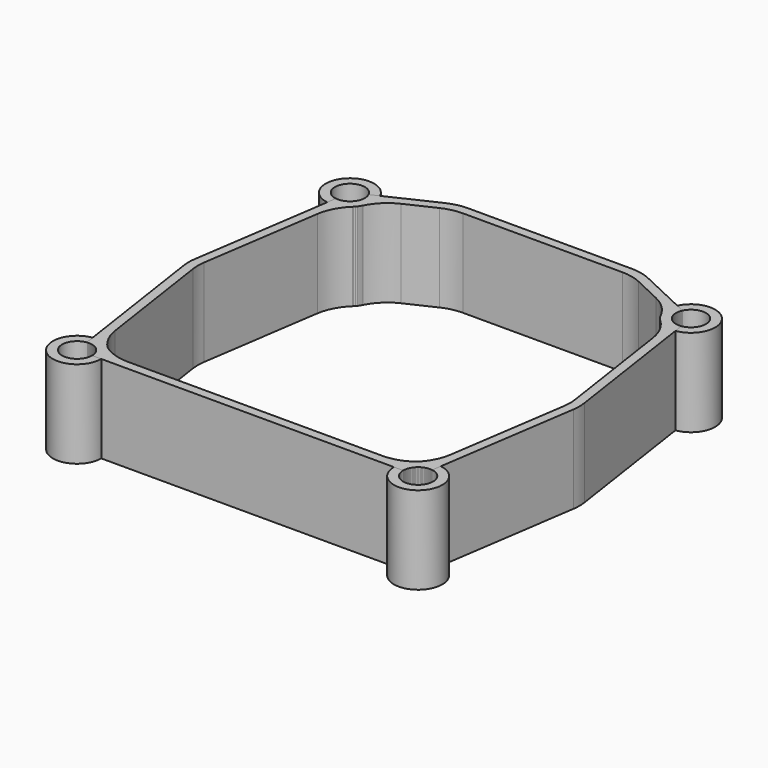
from build123d import *

# Parameters (mm, degrees)
F0_R        = 5.25
F1_DEPTH    = 19
F3_DEPTH    = 19
F4_R        = 3.25
F5_DEPTH    = 25
F7_DEPTH    = 25
F8_T1_DEPTH = 19
F8_T3_DEPTH = 26.4324324324
F8_T5_DEPTH = 30.1768389253


# Not quite as in the source:
# - a fillet or chamfer that OpenCascade refuses, or shapes differently, is made with other operations: its cross-section is extruded or revolved along the edge and cut away or added


with BuildPart() as f1:
    # F0 (on Top) → F1 (new body)
    with BuildSketch(Plane.XY):
        with Locations((-37, 37)):
            Circle(F0_R)
    extrude(amount=F1_DEPTH)


with BuildPart() as f1b:
    # F0 (on Top) → F1, piece 2 (new body)
    with BuildSketch(Plane.XY):
        with Locations((37, 37)):
            Circle(F0_R)
    extrude(amount=F1_DEPTH)


with BuildPart() as f1c:
    # F0 (on Top) → F1, piece 3 (new body)
    with BuildSketch(Plane.XY):
        with Locations((37, -37)):
            Circle(F0_R)
    extrude(amount=F1_DEPTH)


with BuildPart() as f1d:
    # F0 (on Top) → F1, piece 4 (new body)
    with BuildSketch(Plane.XY):
        with Locations((-37, -37)):
            Circle(F0_R)
    extrude(amount=F1_DEPTH)


with BuildPart() as f3:
    # F2 (on Top) → F3 (new body)
    with BuildSketch(Plane.XY):
        Polygon((20, 45), (-20, 45), (-37, 37), (-42.5, 0), (-37, -37), (37, -37), (42.5, 0), (37, 37), align=None)
    extrude(amount=F3_DEPTH)


with BuildPart() as f5_tool:
    # F4 (on Top) → F5 (new body)
    with BuildSketch(Plane.XY):
        with Locations((-37, 37)):
            Circle(F4_R)
        with Locations((37, 37)):
            Circle(F4_R)
        with Locations((37, -37)):
            Circle(F4_R)
        with Locations((-37, -37)):
            Circle(F4_R)
    extrude(amount=F5_DEPTH)


with BuildPart() as f1_1:
    add(f1.part)

    # F5: cut by f5_tool
    add(f5_tool.part, mode=Mode.SUBTRACT)


with BuildPart() as f1b_1:
    add(f1b.part)

    # F5: cut by f5_tool
    add(f5_tool.part, mode=Mode.SUBTRACT)


with BuildPart() as f1c_1:
    add(f1c.part)

    # F5: cut by f5_tool
    add(f5_tool.part, mode=Mode.SUBTRACT)


with BuildPart() as f1d_1:
    add(f1d.part)

    # F5: cut by f5_tool
    add(f5_tool.part, mode=Mode.SUBTRACT)


with BuildPart() as f3_1:
    add(f3.part)

    # F5: cut by f5_tool
    add(f5_tool.part, mode=Mode.SUBTRACT)

    # F6 (on Top) → F7 (cut)
    with BuildSketch(Plane.XY):
        with BuildLine():
            Line((19.552926443, 43), (-19.552926443, 43))
            Line((-19.552926443, 43), (-31.7563055954, 37.25723334))
            ThreePointArc((-31.7563055954, 37.25723334), (-32.7866811629, 33.8678371088), (-35.7354533115, 31.9045685489))
            Line((-35.7354533115, 31.9045685489), (-40.478024312, 0))
            Line((-40.478024312, 0), (-35.7354533115, -31.9045685489))
            ThreePointArc((-35.7354533115, -31.9045685489), (-33.571450675, -33.0241290858), (-32.1458780403, -35))
            Line((-32.1458780403, -35), (32.1458780403, -35))
            ThreePointArc((32.1458780403, -35), (33.571450675, -33.0241290858), (35.7354533115, -31.9045685489))
            Line((35.7354533115, -31.9045685489), (40.478024312, 0))
            Line((40.478024312, 0), (35.7354533115, 31.9045685489))
            ThreePointArc((35.7354533115, 31.9045685489), (32.7866811629, 33.8678371088), (31.7563055954, 37.25723334))
            Line((31.7563055954, 37.25723334), (19.552926443, 43))
        make_face()
    extrude(amount=F7_DEPTH, mode=Mode.SUBTRACT)

    # F8: fillet of radius 10 on 16 edges, made by hand

    # F8_s2 → F8_t1 (join)
    with BuildSketch(Plane.XY):
        with BuildLine():
            ThreePointArc((21.5755290212, 42.048187022), (19.4990867668, 42.7591462285), (17.3175586579, 43))
            Line((17.3175586579, 43), (19.552926443, 43))
            Line((19.552926443, 43), (21.5755290212, 42.048187022))
        make_face()
        with BuildLine():
            ThreePointArc((-17.3175586579, 43), (-19.4990867668, 42.7591462285), (-21.5755290212, 42.048187022))
            Line((-21.5755290212, 42.048187022), (-19.552926443, 43))
            Line((-19.552926443, 43), (-17.3175586579, 43))
        make_face()
        with BuildLine():
            ThreePointArc((-40.2594616371, 1.4703307219), (-40.3681458718, 0), (-40.2594616371, -1.4703307219))
            Line((-40.2594616371, -1.4703307219), (-40.478024312, 0))
            Line((-40.478024312, 0), (-40.2594616371, 1.4703307219))
        make_face()
        with BuildLine():
            ThreePointArc((40.2594616371, -1.4703307219), (40.3681458718, 0), (40.2594616371, 1.4703307219))
            Line((40.2594616371, 1.4703307219), (40.478024312, 0))
            Line((40.478024312, 0), (40.2594616371, -1.4703307219))
        make_face()
        with BuildLine():
            ThreePointArc((-33.3901050909, 33.188024299), (-35.3836316287, 30.5457403999), (-36.405430553, 27.3974489237))
            Line((-36.405430553, 27.3974489237), (-35.7354533115, 31.9045685489))
            ThreePointArc((-35.7354533115, 31.9045685489), (-34.4797103564, 32.3944989293), (-33.3901050909, 33.188024299))
        make_face()
        with BuildLine():
            ThreePointArc((-27.6333696517, 39.19743849), (-30.3537332547, 37.3118526055), (-32.3095636894, 34.6415455874))
            ThreePointArc((-32.3095636894, 34.6415455874), (-31.8636400174, 35.9135810529), (-31.7563055954, 37.25723334))
            Line((-31.7563055954, 37.25723334), (-27.6333696517, 39.19743849))
        make_face()
        with BuildLine():
            ThreePointArc((-33.3901050909, -33.188024299), (-35.3836316287, -30.5457403999), (-36.405430553, -27.3974489237))
            Line((-36.405430553, -27.3974489237), (-35.7354533115, -31.9045685489))
            ThreePointArc((-35.7354533115, -31.9045685489), (-34.4797103564, -32.3944989293), (-33.3901050909, -33.188024299))
        make_face()
        with BuildLine():
            ThreePointArc((-33.7602284039, -32.868852459), (-30.8535476338, -34.452209387), (-27.5892348876, -35))
            Line((-27.5892348876, -35), (-32.1458780403, -35))
            ThreePointArc((-32.1458780403, -35), (-32.8151193944, -33.8299409601), (-33.7602284039, -32.868852459))
        make_face()
        with BuildLine():
            ThreePointArc((36.405430553, 27.3974489237), (35.3836316287, 30.5457403999), (33.3901050909, 33.188024299))
            ThreePointArc((33.3901050909, 33.188024299), (34.4797103564, 32.3944989293), (35.7354533115, 31.9045685489))
            Line((35.7354533115, 31.9045685489), (36.405430553, 27.3974489237))
        make_face()
        with BuildLine():
            ThreePointArc((32.3095636894, 34.6415455874), (30.3537332547, 37.3118526055), (27.6333696517, 39.19743849))
            Line((27.6333696517, 39.19743849), (31.7563055954, 37.25723334))
            ThreePointArc((31.7563055954, 37.25723334), (31.8636400174, 35.9135810529), (32.3095636894, 34.6415455874))
        make_face()
        with BuildLine():
            ThreePointArc((27.5892348876, -35), (30.8535476338, -34.452209387), (33.7602284039, -32.868852459))
            ThreePointArc((33.7602284039, -32.868852459), (32.8151193944, -33.8299409601), (32.1458780403, -35))
            Line((32.1458780403, -35), (27.5892348876, -35))
        make_face()
        with BuildLine():
            ThreePointArc((33.3901050909, -33.188024299), (35.3836316287, -30.5457403999), (36.405430553, -27.3974489237))
            Line((36.405430553, -27.3974489237), (35.7354533115, -31.9045685489))
            ThreePointArc((35.7354533115, -31.9045685489), (34.4797103564, -32.3944989293), (33.3901050909, -33.188024299))
        make_face()
    extrude(amount=F8_T1_DEPTH)

    # F8_s4 → F8_t3 (cut)
    with BuildSketch(Plane.XY.offset(-3.7162162162)):
        with BuildLine():
            ThreePointArc((42.2814373251, 1.4703307219), (42.3901215599, 0), (42.2814373251, -1.4703307219))
            Line((42.2814373251, -1.4703307219), (42.5, 0))
            Line((42.5, 0), (42.2814373251, 1.4703307219))
        make_face()
        with BuildLine():
            ThreePointArc((-42.2814373251, 1.4703307219), (-42.3901215599, 0), (-42.2814373251, -1.4703307219))
            Line((-42.2814373251, -1.4703307219), (-42.5, 0))
            Line((-42.5, 0), (-42.2814373251, 1.4703307219))
        make_face()
    extrude(amount=F8_T3_DEPTH, mode=Mode.SUBTRACT)

    # F8_s6 → F8_t5 (cut)
    with BuildSketch(Plane.XY.offset(-5.5884194627)):
        with BuildLine():
            ThreePointArc((-17.7646322149, 45), (-19.9461603238, 44.7591462285), (-22.0226025782, 44.048187022))
            Line((-22.0226025782, 44.048187022), (-20, 45))
            Line((-20, 45), (-17.7646322149, 45))
        make_face()
        with BuildLine():
            ThreePointArc((17.7646322149, 45), (19.9461603238, 44.7591462285), (22.0226025782, 44.048187022))
            Line((22.0226025782, 44.048187022), (20, 45))
            Line((20, 45), (17.7646322149, 45))
        make_face()
    extrude(amount=F8_T5_DEPTH, mode=Mode.SUBTRACT)


solid = Compound([f1_1.part, f1b_1.part, f1c_1.part, f1d_1.part, f3_1.part])
